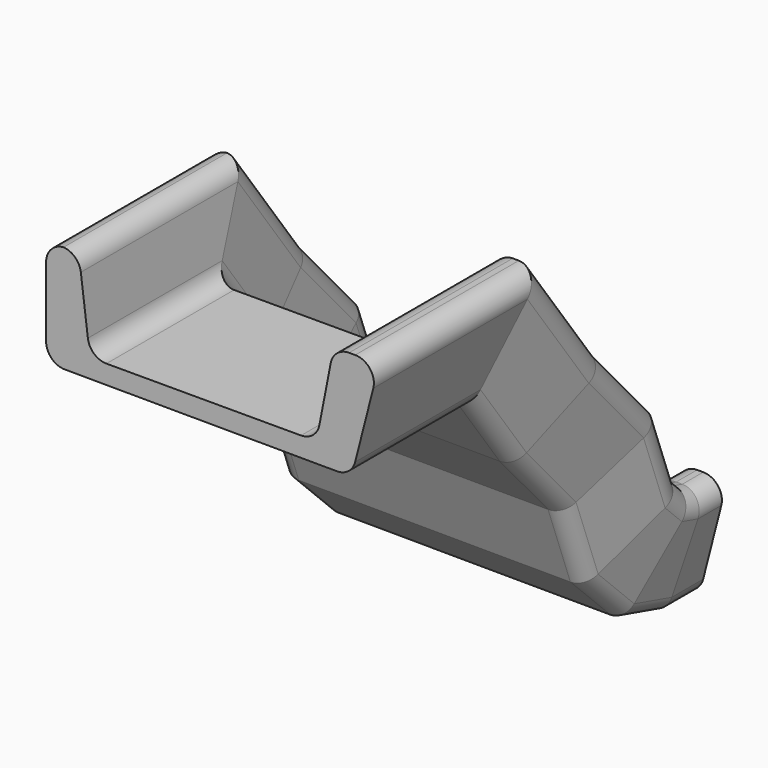
from build123d import *


with BuildPart() as f2:
    # F2: sweep along a path in F1
    with BuildLine(Plane.YZ) as f2_path:
        Line((0, 0), (54.2271062732, 0))
        Line((54.2271062732, 0), (74.3272826076, -27.5529418141))
        Line((74.3272826076, -27.5529418141), (95.5489575863, -51.0973446071))
        Line((95.5489575863, -51.0973446071), (104.9186140299, -76.3795748353))
        Line((104.9186140299, -76.3795748353), (119.5624619722, -90.8030569553))
        Line((119.5624619722, -90.8030569553), (134.8015367985, -95.1338708401))
        Line((134.8015367985, -95.1338708401), (147.8405743837, -95.1338708401))
    # F0 (on Front) → F2 (sweep)
    with BuildSketch(Plane.XZ):
        with BuildLine():
            Line((-51.6746714711, 23.7191500306), (-51.6746714711, 0))
            ThreePointArc((-51.6746714711, 0), (-49.8239963657, -4.4809123505), (-45.350710686, -6.3499466107))
            Line((-45.350710686, -6.3499466107), (47.1804031889, -6.7293887862))
            ThreePointArc((47.1804031889, -6.7293887862), (51.089613293, -5.4037315626), (53.357891469, -1.9549339708))
            Line((53.357891469, -1.9549339708), (59.5256559013, 22.1268726525))
            ThreePointArc((59.5256559013, 22.1268726525), (58.3905238566, 27.5958286572), (53.374206836, 30.0523644478))
            Line((53.374206836, 30.0523644478), (51.2866688171, 30.0523644478))
            ThreePointArc((51.2866688171, 30.0523644478), (47.2485796403, 28.6030109154), (45.0538349714, 24.9165646999))
            Line((45.0538349714, 24.9165646999), (41.2004016239, 5.1357997479))
            ThreePointArc((41.2004016239, 5.1357997479), (39.005656955, 1.4493535324), (34.9675677782, 0))
            Line((34.9675677782, 0), (-31.172045563, 0))
            ThreePointArc((-31.172045563, 0), (-35.3717492022, 1.587123837), (-37.472098588, 5.5551214666))
            Line((-37.472098588, 5.5551214666), (-39.8641464341, 24.514028564))
            ThreePointArc((-39.8641464341, 24.514028564), (-41.8092828653, 28.3405352625), (-45.7444354651, 30.0552606822))
            ThreePointArc((-45.7444354651, 30.0552606822), (-49.9608337505, 28.0583319027), (-51.6746714711, 23.7191500306))
        make_face()
    sweep(path=f2_path.line, transition=Transition.RIGHT)


solid = f2.part
